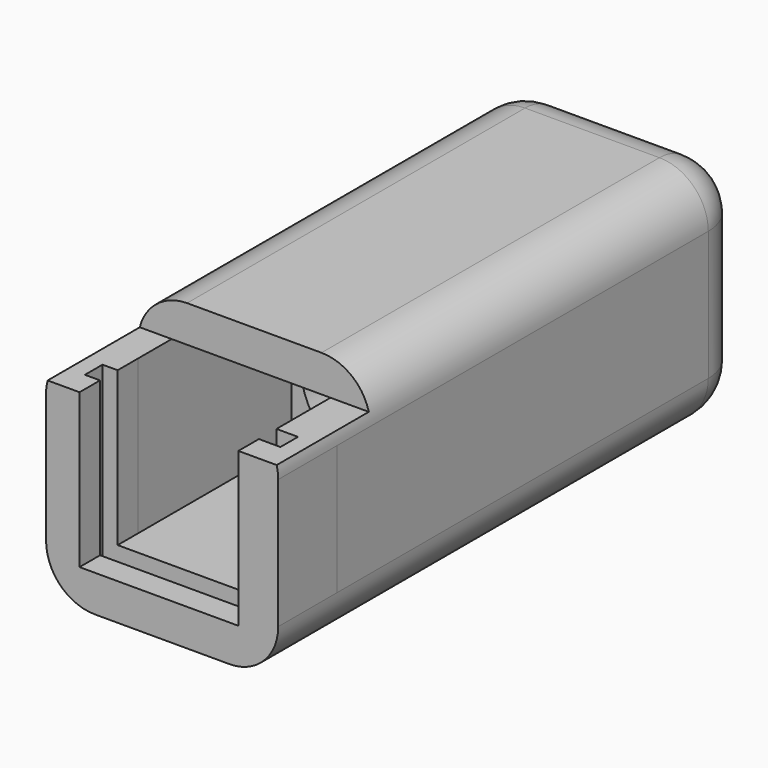
from build123d import *

# Parameters (mm, degrees)
F0_W         = 1.3692331631
F0_H         = 7.834737435
F0_W_2       = 6.5
F0_H_2       = 0.9
F0_W_3       = 0.6192331631
F0_H_3       = 1.05
F0_H_4       = 13.165262565
F0_W_4       = 0.8807668369
F0_W_5       = 1.6307668369
F1_DEPTH     = 0.9
F2_DEPTH     = 1.5
F3_DEPTH     = 7.8
F5_W         = 9.5
F5_H         = 19.2867757659
F6_DEPTH     = 1.5
F7_R         = 3
F8_DEPTH     = 22.501
F9_T1_DEPTH  = 5.3
F9_T3_DEPTH  = 5.5
F9_T5_DEPTH  = 22.2867757659
F9_T7_DEPTH  = 27
F9_S11_W     = 2
F9_S11_H     = 2
F9_T12_DEPTH = 2
F9_S17_W     = 2
F9_S17_H     = 2
F9_T18_DEPTH = 2
F9_S23_W     = 2
F9_S23_H     = 2
F9_T24_DEPTH = 2
F9_S29_W     = 2
F9_S29_H     = 2
F9_T30_DEPTH = 2


# Not quite as in the source:
# - a fillet or chamfer that OpenCascade refuses, or shapes differently, is made with other operations: its cross-section is extruded or revolved along the edge and cut away or added
# - a feature names something its author has since deleted; it is built from what else it names


with BuildPart() as f1:
    # F0 (on Top) → F1 (new body)
    with BuildSketch(Plane.XY):
        Polygon((-4.75, 1.5), (-4.75, -1.5), (-3.3807668369, -1.5), (-3.3807668369, -0.45), (-4, -0.45), (-4, 0.45), (-3.3807668369, 0.45), (-3.3807668369, 1.5), align=None)
        Polygon((-3.3807668369, -0.45), (-3.3807668369, -1.5), (-3.1192331631, -1.5), (3.1192331631, -1.5), (3.1192331631, -0.45), align=None)
        with Locations((-4.0653834185, 5.4173687175)):
            Rectangle(F0_W, F0_H)
        with Locations((-0.1307668369, 0)):
            Rectangle(F0_W_2, F0_H_2)
        with Locations((-3.6903834185, 0)):
            Rectangle(F0_W_3, F0_H_2)
        with Locations((-0.1307668369, 5.4173687175)):
            Rectangle(F0_W_2, F0_H)
        with Locations((-0.1307668369, 0.975)):
            Rectangle(F0_W_2, F0_H_3)
        with Locations((-4.0653834185, 15.9173687175)):
            Rectangle(F0_W, F0_H_4)
        Polygon((3.1192331631, -0.45), (3.1192331631, -1.5), (3.3807668369, -1.5), (4.75, -1.5), (4.75, 1.5), (3.1192331631, 1.5), (3.1192331631, 0.45), (4, 0.45), (4, -0.45), align=None)
        with Locations((3.5596165815, 0)):
            Rectangle(F0_W_4, F0_H_2)
        with Locations((3.9346165815, 5.4173687175)):
            Rectangle(F0_W_5, F0_H)
        with Locations((-0.1307668369, 15.9173687175)):
            Rectangle(F0_W_2, F0_H_4)
        with Locations((3.9346165815, 15.9173687175)):
            Rectangle(F0_W_5, F0_H_4)
    extrude(amount=F1_DEPTH)

    # F0 (on Top) → F2 (join)
    with BuildSketch(Plane.XY):
        Polygon((-3.3807668369, -0.45), (-3.3807668369, -1.5), (-3.1192331631, -1.5), (3.1192331631, -1.5), (3.1192331631, -0.45), align=None)
        Polygon((3.1192331631, -0.45), (3.1192331631, -1.5), (3.3807668369, -1.5), (4.75, -1.5), (4.75, 1.5), (3.1192331631, 1.5), (3.1192331631, 0.45), (4, 0.45), (4, -0.45), align=None)
        Polygon((-4.75, 1.5), (-4.75, -1.5), (-3.3807668369, -1.5), (-3.3807668369, -0.45), (-4, -0.45), (-4, 0.45), (-3.3807668369, 0.45), (-3.3807668369, 1.5), align=None)
        with Locations((-0.1307668369, 0.975)):
            Rectangle(F0_W_2, F0_H_3)
        with Locations((-4.0653834185, 5.4173687175)):
            Rectangle(F0_W, F0_H)
        with Locations((3.9346165815, 5.4173687175)):
            Rectangle(F0_W_5, F0_H)
        with Locations((-0.1307668369, 5.4173687175)):
            Rectangle(F0_W_2, F0_H)
        with Locations((-4.0653834185, 15.9173687175)):
            Rectangle(F0_W, F0_H_4)
        with Locations((-0.1307668369, 15.9173687175)):
            Rectangle(F0_W_2, F0_H_4)
        with Locations((3.9346165815, 15.9173687175)):
            Rectangle(F0_W_5, F0_H_4)
    extrude(amount=F2_DEPTH)

    # F0 (on Top) → F3 (join)
    with BuildSketch(Plane.XY):
        Polygon((-4.75, 1.5), (-4.75, -1.5), (-3.3807668369, -1.5), (-3.3807668369, -0.45), (-4, -0.45), (-4, 0.45), (-3.3807668369, 0.45), (-3.3807668369, 1.5), align=None)
        Polygon((3.1192331631, -0.45), (3.1192331631, -1.5), (3.3807668369, -1.5), (4.75, -1.5), (4.75, 1.5), (3.1192331631, 1.5), (3.1192331631, 0.45), (4, 0.45), (4, -0.45), align=None)
        with Locations((-4.0653834185, 5.4173687175)):
            Rectangle(F0_W, F0_H)
        with Locations((3.9346165815, 5.4173687175)):
            Rectangle(F0_W_5, F0_H)
        with Locations((-4.0653834185, 15.9173687175)):
            Rectangle(F0_W, F0_H_4)
        with Locations((-0.1307668369, 15.9173687175)):
            Rectangle(F0_W_2, F0_H_4)
        with Locations((3.9346165815, 15.9173687175)):
            Rectangle(F0_W_5, F0_H_4)
    extrude(amount=F3_DEPTH)

    # F5 (on offset) → F6 (join)
    with BuildSketch(Plane.XY.offset(7.8)):
        with Locations((0, 12.856612117)):
            Rectangle(F5_W, F5_H)
    extrude(amount=F6_DEPTH)

    # F7 (on Front) → F8 (cut, through all)
    with BuildSketch(Plane.XZ):
        with Locations((0, 4.5)):
            Circle(F7_R)
    extrude(amount=-F8_DEPTH, mode=Mode.SUBTRACT)

    # F9: fillet of radius 2 on 8 edges, made by hand

    # F9_s2 → F9_t1 (cut)
    with BuildSketch(Plane.XY.offset(2)):
        with BuildLine():
            ThreePointArc((4.75, 20.5), (4.1642135624, 21.9142135624), (2.75, 22.5))
            Line((2.75, 22.5), (4.75, 22.5))
            Line((4.75, 22.5), (4.75, 20.5))
        make_face()
        with BuildLine():
            ThreePointArc((-4.75, 20.5), (-4.1642135624, 21.9142135624), (-2.75, 22.5))
            Line((-2.75, 22.5), (-4.75, 22.5))
            Line((-4.75, 22.5), (-4.75, 20.5))
        make_face()
    extrude(amount=F9_T1_DEPTH, mode=Mode.SUBTRACT)

    # F9_s4 → F9_t3 (cut)
    with BuildSketch(Plane.YZ.offset(-2.75)):
        with BuildLine():
            ThreePointArc((20.5, 9.3), (21.9142135624, 8.7142135624), (22.5, 7.3))
            Line((22.5, 7.3), (22.5, 9.3))
            Line((22.5, 9.3), (20.5, 9.3))
        make_face()
        with BuildLine():
            ThreePointArc((20.5, 0), (21.9142135624, 0.5857864376), (22.5, 2))
            Line((22.5, 2), (22.5, 0))
            Line((22.5, 0), (20.5, 0))
        make_face()
    extrude(amount=F9_T3_DEPTH, mode=Mode.SUBTRACT)

    # F9_s6 → F9_t5 (cut)
    with BuildSketch(Plane.XZ.offset(-20.5)):
        with BuildLine():
            ThreePointArc((4.75, 7.3), (4.1642135624, 8.7142135624), (2.75, 9.3))
            Line((2.75, 9.3), (4.75, 9.3))
            Line((4.75, 9.3), (4.75, 7.3))
        make_face()
        with BuildLine():
            ThreePointArc((-4.75, 7.3), (-4.1642135624, 8.7142135624), (-2.75, 9.3))
            Line((-2.75, 9.3), (-4.75, 9.3))
            Line((-4.75, 9.3), (-4.75, 7.3))
        make_face()
    extrude(amount=F9_T5_DEPTH, mode=Mode.SUBTRACT)

    # F9_s8 → F9_t7 (cut)
    with BuildSketch(Plane.XZ.offset(-20.5)):
        with BuildLine():
            ThreePointArc((2.75, 0), (4.1642135624, 0.5857864376), (4.75, 2))
            Line((4.75, 2), (4.75, 0))
            Line((4.75, 0), (2.75, 0))
        make_face()
        with BuildLine():
            ThreePointArc((-4.75, 2), (-4.1642135624, 0.5857864376), (-2.75, 0))
            Line((-2.75, 0), (-4.75, 0))
            Line((-4.75, 0), (-4.75, 2))
        make_face()
    extrude(amount=F9_T7_DEPTH, mode=Mode.SUBTRACT)


with BuildPart() as f9_tool10:
    # F9_s11 → F9_t12 (new body)
    with BuildSketch(Plane.YZ.offset(2.75)):
        with Locations((21.5, 8.3)):
            Rectangle(F9_S11_W, F9_S11_H)
    extrude(amount=F9_T12_DEPTH)

    # F9_s13 → F9_t14 (revolve, cut)
    with BuildSketch(Plane(origin=(2.75, 20.5, 7.3), x_dir=(0, -0.7071067812, -0.7071067812), z_dir=(0, -0.7071067812, 0.7071067812))):
        with BuildLine():
            ThreePointArc((0, -2), (2, 0), (0, 2))
            Line((0, 2), (0, -2))
        make_face()
    revolve(axis=Axis((2.75, 20.5, 7.3), (1, 0, 0)), mode=Mode.SUBTRACT)


with BuildPart() as f1_1:
    add(f1.part)

    # F9_t9: cut F9_tool10
    add(f9_tool10.part, mode=Mode.SUBTRACT)


with BuildPart() as f9_tool16:
    # F9_s17 → F9_t18 (new body)
    with BuildSketch(Plane.XY.offset(2)):
        with Locations((3.75, 21.5)):
            Rectangle(F9_S17_W, F9_S17_H)
    extrude(amount=-F9_T18_DEPTH)

    # F9_s19 → F9_t20 (revolve, cut)
    with BuildSketch(Plane(origin=(2.75, 20.5, 2), x_dir=(-0.7071067812, -0.7071067812, 0), z_dir=(0.7071067812, -0.7071067812, 0))):
        with BuildLine():
            ThreePointArc((0, -2), (2, 0), (0, 2))
            Line((0, 2), (0, -2))
        make_face()
    revolve(axis=Axis((2.75, 20.5, 2), (0, 0, -1)), mode=Mode.SUBTRACT)


with BuildPart() as f1_2:
    add(f1_1.part)

    # F9_t15: cut F9_tool16
    add(f9_tool16.part, mode=Mode.SUBTRACT)


with BuildPart() as f9_tool22:
    # F9_s23 → F9_t24 (new body)
    with BuildSketch(Plane.YZ.offset(-2.75)):
        with Locations((21.5, 8.3)):
            Rectangle(F9_S23_W, F9_S23_H)
    extrude(amount=-F9_T24_DEPTH)

    # F9_s25 → F9_t26 (revolve, cut)
    with BuildSketch(Plane(origin=(-2.75, 20.5, 7.3), x_dir=(0, -0.7071067812, -0.7071067812), z_dir=(0, 0.7071067812, -0.7071067812))):
        with BuildLine():
            ThreePointArc((0, -2), (2, 0), (0, 2))
            Line((0, 2), (0, -2))
        make_face()
    revolve(axis=Axis((-2.75, 20.5, 7.3), (-1, 0, 0)), mode=Mode.SUBTRACT)


with BuildPart() as f1_3:
    add(f1_2.part)

    # F9_t21: cut F9_tool22
    add(f9_tool22.part, mode=Mode.SUBTRACT)


with BuildPart() as f9_tool28:
    # F9_s29 → F9_t30 (new body)
    with BuildSketch(Plane.YZ.offset(-2.75)):
        with Locations((21.5, 1)):
            Rectangle(F9_S29_W, F9_S29_H)
    extrude(amount=-F9_T30_DEPTH)

    # F9_s31 → F9_t32 (revolve, cut)
    with BuildSketch(Plane(origin=(-2.75, 20.5, 2), x_dir=(0, -0.7071067812, 0.7071067812), z_dir=(0, -0.7071067812, -0.7071067812))):
        with BuildLine():
            ThreePointArc((0, -2), (2, 0), (0, 2))
            Line((0, 2), (0, -2))
        make_face()
    revolve(axis=Axis((-2.75, 20.5, 2), (-1, 0, 0)), mode=Mode.SUBTRACT)


with BuildPart() as f1_4:
    add(f1_3.part)

    # F9_t27: cut F9_tool28
    add(f9_tool28.part, mode=Mode.SUBTRACT)


solid = f1_4.part
